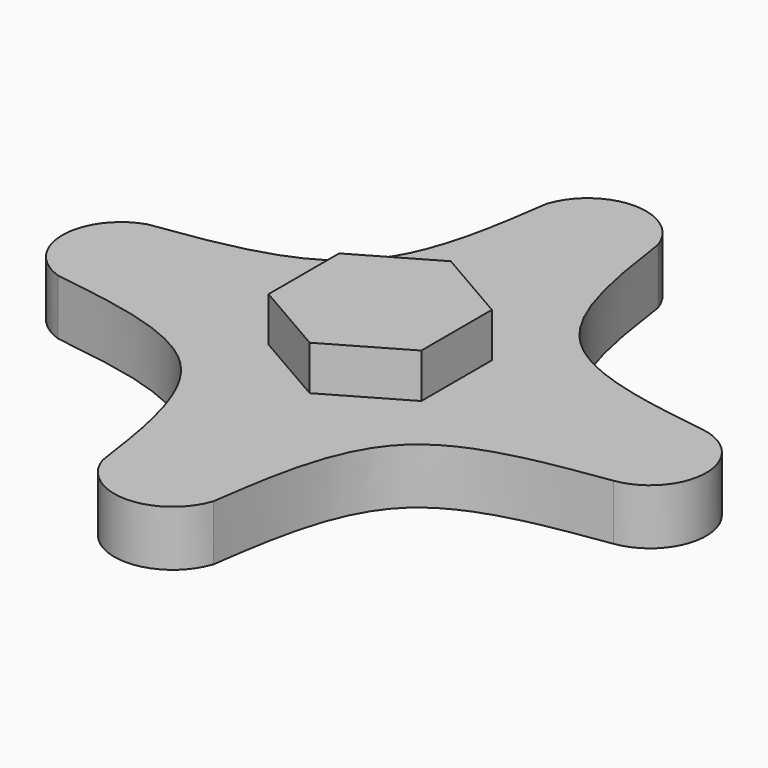
from build123d import *

# Parameters (mm, degrees)
F1_DEPTH     = 5
F3_DEPTH     = 4
F4_TEXT_SIZE = 8.3333333333
F5_DEPTH     = 1


# Not quite as in the source:
# - Text() gives the source's letters only with a copy of the font that has no kerning and outlines rounded to 1/6400 em; it was checked with that copy


with BuildPart() as f1:
    # F0 (on Top) → F1 (new body)
    with BuildSketch(Plane.XY):
        with BuildLine():
            ThreePointArc((5, 25), (0, 28.6037961003), (-5, 25))
            add(Edge.make_bspline(
                [(-25, 5), (-19.1666666667, 5.8333333333), (-7.5, 7.5), (-5.8333333333, 19.1666666667), (-5, 25)],
                knots=[0, 0, 0, 0, 0.5, 1, 1, 1, 1], degree=3))
            ThreePointArc((-25, 5), (-28.6037961003, 0), (-25, -5))
            add(Edge.make_bspline(
                [(-25, -5), (-19.1666666667, -5.8333333333), (-7.5, -7.5), (-5.8333333333, -19.1666666667), (-5, -25)],
                knots=[0, 0, 0, 0, 0.5, 1, 1, 1, 1], degree=3))
            ThreePointArc((-5, -25), (0, -28.6037961003), (5, -25))
            add(Edge.make_bspline(
                [(5, -25), (5.8350479613, -19.1710743293), (7.4979427005, -7.481622601), (19.1690666377, -5.8656804687), (25, -5)],
                knots=[0, 0, 0, 0, 0.5, 1, 1, 1, 1], degree=3))
            ThreePointArc((25, -5), (29.3364770085, 0), (25, 5))
            add(Edge.make_bspline(
                [(5, 25), (5.8333333333, 19.1666666667), (7.5, 7.5), (19.1666666667, 5.8333333333), (25, 5)],
                knots=[0, 0, 0, 0, 0.5, 1, 1, 1, 1], degree=3))
        make_face()
    extrude(amount=F1_DEPTH)

    # F2 (on face) → F3 (join)
    with BuildSketch(Plane.XY.offset(5)):
        Polygon((6.875, 3.9692831007), (0, 7.9385662014), (-6.875, 3.9692831007), (-6.875, -3.9692831007), (0, -7.9385662014), (6.875, -3.9692831007), align=None)
    extrude(amount=F3_DEPTH)

    # F4 (on face) → F5 (cut)
    with BuildSketch(Plane(origin=(0, 0, 0), x_dir=(1, 0, 0), z_dir=(0, 0, -1))):
        with Locations((-26.5, -3)):
            Text('Mad Engineer', F4_TEXT_SIZE, font='Open Sans', text_align=(TextAlign.LEFT, TextAlign.BOTTOM))
    extrude(amount=-F5_DEPTH, mode=Mode.SUBTRACT)


solid = f1.part
